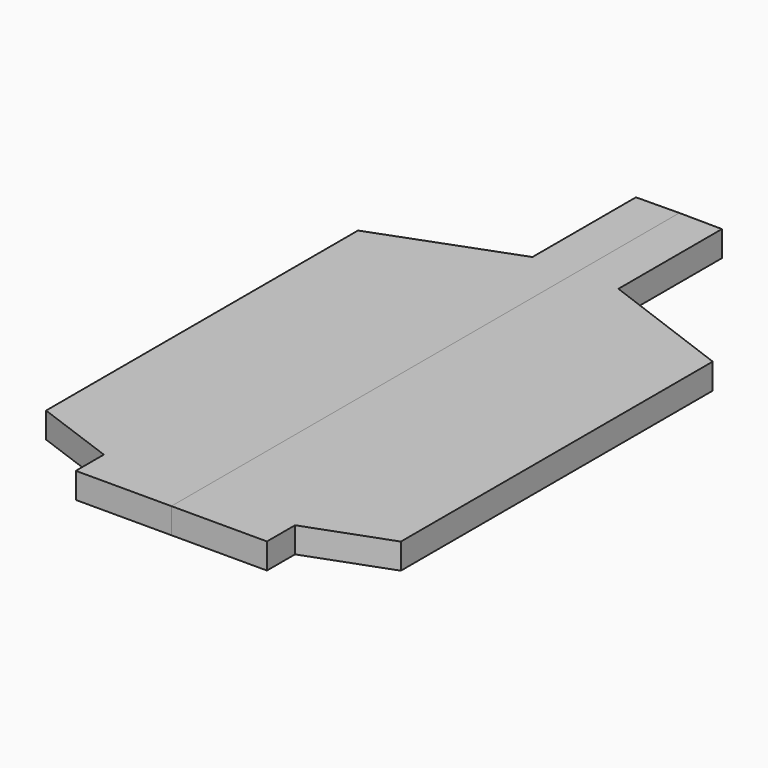
from build123d import *

# Parameters (mm, degrees)
F1_DEPTH = 5


# Not quite as in the source:
# - a pattern or mirror of a feature is missing from the dataset's text; its kind, count and spacing are read off the source's solid
# - a feature names something its author has since deleted; it is built from what else it names


with BuildPart() as f1:
    # F0 (on Top) → F1 (new body)
    with BuildSketch(Plane.XY):
        Polygon((0, 46.6559864581), (-8.3835506812, 46.5571954846), (-8.3835506812, 21.3251467794), (-34.5923192799, 11.5579040721), (-34.5923192799, -64.463801682), (-18.6391565949, -70.3241527081), (-18.6391565949, -77.1612226963), (0, -77.1612226963), align=None)
    extrude(amount=F1_DEPTH)


with BuildPart() as f1_copies_1:
    # F1_copies: instance of F1
    add(f1.part.mirror(Plane(origin=(0, 0, 0), x_dir=(0, 0, 1), z_dir=(1, 0, 0))))


solid = Compound([f1.part, f1_copies_1.part])
